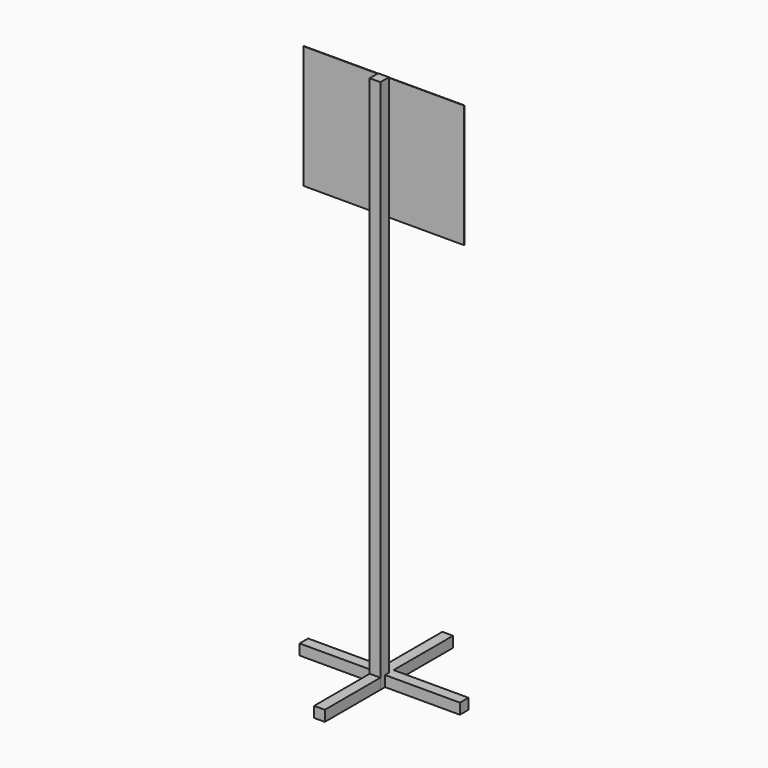
from build123d import *

# Parameters (mm, degrees)
F0_W     = 311.0204081633
F0_H     = 238.4489795918
F1_DEPTH = 1
F2_W     = 20.7346938776
F2_H     = 1.0367346939
F3_DEPTH = 20.7346938776
F5_W     = 20.7346938776
F5_H     = 20.7346938776
F6_DEPTH = 155.5102040816
F7_W     = 20.7346938776
F7_H     = 20.7346938776
F8_DEPTH = 155.5102040816
F4_W     = 20.7346938776
F4_H     = 20.7346938776
F9_DEPTH = 1036.7346938776


# Not quite as in the source:
# - the program builds the solid bodies; features that only make, move or delete a surface that nothing else refers to are left out


with BuildPart() as f1:
    # F0 (on Front) → F1 (new body)
    with BuildSketch(Plane.XZ):
        with Locations((0.3589130938, 13.0331495404)):
            Rectangle(F0_W, F0_H)
    extrude(amount=F1_DEPTH)

    # F2 (on face) → F3 (join)
    with BuildSketch(Plane.XZ.offset(1)):
        with Locations((0, 132.7760066833)):
            Rectangle(F2_W, F2_H)
    extrude(amount=F3_DEPTH)


with BuildPart() as f6:
    # F5 (on face) → F6 (new body, symmetric)
    with BuildSketch(Plane.XZ.offset(1)):
        with Locations((0, -894.1097076024)):
            Rectangle(F5_W, F5_H)
    extrude(amount=F6_DEPTH, both=True)

    # F7 (on Right) → F8 (join, symmetric)
    with BuildSketch(Plane.YZ):
        with Locations((0, -894.1097076024)):
            Rectangle(F7_W, F7_H)
    extrude(amount=F8_DEPTH, both=True)


with BuildPart() as f9:
    # F4 (on face) → F9 (new body)
    with BuildSketch(Plane(origin=(0, 0, 132.2576393363), x_dir=(1, 0, 0), z_dir=(0, 0, -1))):
        with Locations((0, 11.3673469388)):
            Rectangle(F4_W, F4_H)
    extrude(amount=F9_DEPTH)


solid = Compound([f1.part, f6.part, f9.part])
